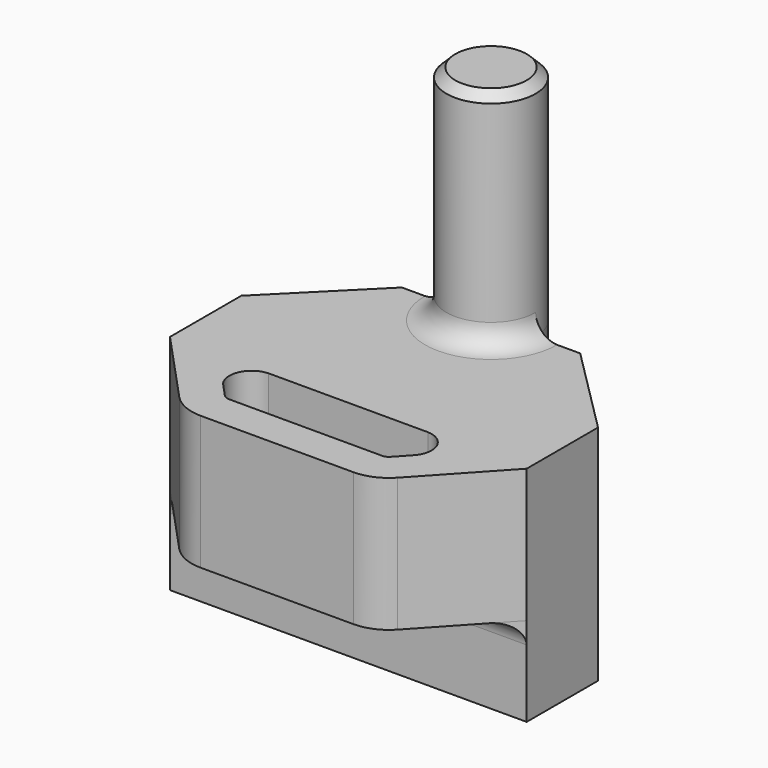
from build123d import *

# Parameters (mm, degrees)
F1_DEPTH     = 5
F2_DEPTH     = 10
F3_SIZE      = 0.2
F5_DEPTH     = 3
F6_T1_DEPTH  = 3
F6_T6_DEPTH  = 2.3418509092
F6_T12_DEPTH = 2.3418509092
F6_T16_ANGLE = 180
F6_T21_DEPTH = 2.3418509092
F6_T25_DEPTH = 5.8592538582
F6_T33_DEPTH = 5.8592538582
F6_T38_DEPTH = 2.3418509092


# Not quite as in the source:
# - a fillet or chamfer that OpenCascade refuses, or shapes differently, is made with other operations: its cross-section is extruded or revolved along the edge and cut away or added


with BuildPart() as f1:
    # F0 (on Top) → F1 (new body)
    with BuildSketch(Plane.XY):
        with BuildLine():
            Line((0, 2), (0, 0))
            Line((0, 0), (8, 0))
            Line((8, 0), (8, 2))
            Line((8, 2), (6, 4))
            Line((6, 4), (5, 4))
            ThreePointArc((5, 4), (4, 3), (3, 4))
            Line((3, 4), (2, 4))
            Line((2, 4), (0, 2))
        make_face()
        with BuildLine():
            ThreePointArc((5, 4), (4, 5), (3, 4))
            Line((3, 4), (5, 4))
        make_face()
        with BuildLine():
            Line((5, 4), (3, 4))
            ThreePointArc((3, 4), (4, 3), (5, 4))
        make_face()
    extrude(amount=F1_DEPTH)

    # F0 (on Top) → F2 (join)
    with BuildSketch(Plane.XY):
        with BuildLine():
            ThreePointArc((5, 4), (4, 5), (3, 4))
            Line((3, 4), (5, 4))
        make_face()
        with BuildLine():
            Line((5, 4), (3, 4))
            ThreePointArc((3, 4), (4, 3), (5, 4))
        make_face()
    extrude(amount=F2_DEPTH)

    # F3
    f3_edges = [f1.edges().sort_by_distance(p)[0] for p in [
        (5, 4, 10),
    ]]
    chamfer(f3_edges, length=F3_SIZE)

    # F4 (on face) → F5 (join)
    with BuildSketch(Plane.XY.offset(5)):
        with BuildLine():
            Line((1.0894362964, 0), (0, 0))
            Line((0, 0), (1.5518551177, -1.6787983581))
            ThreePointArc((1.5518551177, -1.6787983581), (1.8854295116, -1.9161873057), (2.286179834, -2))
            Line((2.286179834, -2), (5.713820166, -2))
            ThreePointArc((5.713820166, -2), (6.1145704884, -1.9161873057), (6.4481448823, -1.6787983581))
            Line((6.4481448823, -1.6787983581), (8, 0))
            Line((8, 0), (6.9105637036, 0))
            Line((6.9105637036, 0), (5.8606851097, -1.1357596721))
            ThreePointArc((5.8606851097, -1.1357596721), (5.7939702307, -1.1832374617), (5.713820166, -1.2000000007))
            Line((5.713820166, -1.2000000007), (2.286179834, -1.2000000007))
            ThreePointArc((2.286179834, -1.2000000007), (2.2060297693, -1.1832374617), (2.1393148903, -1.1357596721))
            Line((2.1393148903, -1.1357596721), (1.0894362964, 0))
        make_face()
    extrude(amount=-F5_DEPTH)

    # F6: fillet of radius 0.5 on 5 edges, made by hand

    # F6_s2 → F6_t1 (join)
    with BuildSketch(Plane.XY.offset(2)):
        with BuildLine():
            ThreePointArc((5.7668622302, 0.0004), (6.2255674394, -0.2996248388), (6.1345147512, -0.8401197793))
            Line((6.1345147512, -0.8401197793), (6.1712800033, -0.8741050071))
            ThreePointArc((6.1712800033, -0.8741050071), (6.5591576145, -0.4539093578), (6.9473289557, -0.0339852278))
            Line((6.9473289557, -0.0339852278), (6.9105637036, 0.0500667501))
            ThreePointArc((6.9105637036, 0.0500667501), (6.3387129669, 0.0500667501), (5.7668622302, 0.0504667501))
            Line((5.7668622302, 0.0504667501), (5.7668622302, 0.0004))
        make_face()
        with BuildLine():
            ThreePointArc((2.2331377698, 0.0004), (1.7744325606, -0.2996248388), (1.8654852488, -0.8401197793))
            Line((1.8654852488, -0.8401197793), (1.8287199967, -0.8741050071))
            ThreePointArc((1.8287199967, -0.8741050071), (1.4408423855, -0.4539093578), (1.0526710443, -0.0339852278))
            Line((1.0526710443, -0.0339852278), (1.0894362964, 0.0500667501))
            ThreePointArc((1.0894362964, 0.0500667501), (1.6612870331, 0.0500667501), (2.2331377698, 0.0504667501))
            Line((2.2331377698, 0.0504667501), (2.2331377698, 0.0004))
        make_face()
    extrude(amount=F6_T1_DEPTH)


with BuildPart() as f6_tool4:
    # F6_s5 → F6_t6 (new body)
    with BuildSketch(Plane.YZ.offset(8)):
        with BuildLine():
            ThreePointArc((0.0004, 1.4990343146), (-0.1464466094, 1.8535533906), (-0.5009656854, 2.0004))
            Line((-0.5009656854, 2.0004), (-0.5009656854, 2.0505365685))
            ThreePointArc((-0.5009656854, 2.0505365685), (-0.2504828427, 2.0501365685), (0, 2.0501365685))
            Line((0, 2.0501365685), (0.0501365685, 2))
            ThreePointArc((0.0501365685, 2), (0.0501365685, 1.7495171573), (0.0505365685, 1.4990343146))
            Line((0.0505365685, 1.4990343146), (0.0004, 1.4990343146))
        make_face()
    extrude(amount=-F6_T6_DEPTH)

    split(bisect_by=Plane(origin=(4.3138623121, -3.9876672942, 0), x_dir=(0, 0, 1), z_dir=(-0.7343247163, 0.6787983581, 0)), keep=Keep.TOP)

    split(bisect_by=Plane(origin=(3.7264025395, -3.4446286081, 0), x_dir=(0, 0, 1), z_dir=(0.7343247163, -0.6787983581, 0)), keep=Keep.TOP)


with BuildPart() as f1_1:
    add(f1.part)

    # F6_t3: union F6_tool4
    add(f6_tool4.part)


with BuildPart() as f6_tool10:
    # F6_s11 → F6_t12 (new body)
    with BuildSketch(Plane.YZ.offset(2.3418509092)):
        with BuildLine():
            ThreePointArc((0.0004, 1.4990343146), (-0.1464466094, 1.8535533906), (-0.5009656854, 2.0004))
            Line((-0.5009656854, 2.0004), (-0.5009656854, 2.0505365685))
            ThreePointArc((-0.5009656854, 2.0505365685), (-0.2504828427, 2.0501365685), (0, 2.0501365685))
            Line((0, 2.0501365685), (0.0501365685, 2))
            ThreePointArc((0.0501365685, 2), (0.0501365685, 1.7495171573), (0.0505365685, 1.4990343146))
            Line((0.0505365685, 1.4990343146), (0.0004, 1.4990343146))
        make_face()
    extrude(amount=-F6_T12_DEPTH)

    split(bisect_by=Plane(origin=(0, 0, 0), x_dir=(0, 0, 1), z_dir=(0.7343247163, 0.6787983581, 0)), keep=Keep.TOP)

    split(bisect_by=Plane(origin=(0.5874597726, 0.543038686, 0), x_dir=(0, 0, 1), z_dir=(-0.7343247163, -0.6787983581, 0)), keep=Keep.TOP)


with BuildPart() as f1_2:
    add(f1_1.part)

    # F6_t9: union F6_tool10
    add(f6_tool10.part)

    # F6_s15 → F6_t16 (revolve)
    with BuildSketch(Plane.XZ.offset(-4)):
        with BuildLine():
            ThreePointArc((4.9996, 5.5009656854), (5.1464466094, 5.1464466094), (5.5009656854, 4.9996))
            Line((5.5009656854, 4.9996), (5.5009656854, 4.9494634315))
            ThreePointArc((5.5009656854, 4.9494634315), (5.2504828427, 4.9498634315), (5, 4.9498634315))
            Line((5, 4.9498634315), (4.9498634315, 5))
            ThreePointArc((4.9498634315, 5), (4.9498634315, 5.2504828427), (4.9494634315, 5.5009656854))
            Line((4.9494634315, 5.5009656854), (4.9996, 5.5009656854))
        make_face()
    revolve(axis=Axis((4, 4, 5), (0, 0, -1)), revolution_arc=F6_T16_ANGLE)


with BuildPart() as f6_tool19:
    # F6_s20 → F6_t21 (new body)
    with BuildSketch(Plane.YZ.offset(8)):
        with BuildLine():
            ThreePointArc((0.0004, 1.4990343146), (-0.1464466094, 1.8535533906), (-0.5009656854, 2.0004))
            Line((-0.5009656854, 2.0004), (-0.5009656854, 2.0505365685))
            ThreePointArc((-0.5009656854, 2.0505365685), (-0.2504828427, 2.0501365685), (0, 2.0501365685))
            Line((0, 2.0501365685), (0.0501365685, 2))
            ThreePointArc((0.0501365685, 2), (0.0501365685, 1.7495171573), (0.0505365685, 1.4990343146))
            Line((0.0505365685, 1.4990343146), (0.0004, 1.4990343146))
        make_face()
    extrude(amount=-F6_T21_DEPTH)

    split(bisect_by=Plane(origin=(3.7264025395, -3.4446286081, 0), x_dir=(0, 0, 1), z_dir=(-0.7343247163, 0.6787983581, 0)), keep=Keep.TOP)


with BuildPart() as f6_tool23:
    # F6_s24 → F6_t25 (new body)
    with BuildSketch(Plane.XY.offset(5)):
        with BuildLine():
            ThreePointArc((5.7668622302, 0.0004), (6.2255674394, -0.2996248388), (6.1345147512, -0.8401197793))
            Line((6.1345147512, -0.8401197793), (6.1712800033, -0.8741050071))
            ThreePointArc((6.1712800033, -0.8741050071), (6.5591576145, -0.4539093578), (6.9473289557, -0.0339852278))
            Line((6.9473289557, -0.0339852278), (6.9105637036, 0.0500667501))
            ThreePointArc((6.9105637036, 0.0500667501), (6.3387129669, 0.0500667501), (5.7668622302, 0.0504667501))
            Line((5.7668622302, 0.0504667501), (5.7668622302, 0.0004))
        make_face()
    extrude(amount=-F6_T25_DEPTH)

    split(bisect_by=Plane.XY, keep=Keep.TOP)

    split(bisect_by=Plane.XY.offset(2), keep=Keep.BOTTOM)


with BuildPart() as f6_tool19_1:
    add(f6_tool19.part)

    # F6_t28: intersect F6_tool23
    add(f6_tool23.part, mode=Mode.INTERSECT)


with BuildPart() as f1_3:
    add(f1_2.part)

    # F6_t17: union F6_tool19
    add(f6_tool19_1.part)


with BuildPart() as f6_tool31:
    # F6_s32 → F6_t33 (new body)
    with BuildSketch(Plane.XY.offset(5)):
        with BuildLine():
            ThreePointArc((2.2331377698, 0.0004), (1.7744325606, -0.2996248388), (1.8654852488, -0.8401197793))
            Line((1.8654852488, -0.8401197793), (1.8287199967, -0.8741050071))
            ThreePointArc((1.8287199967, -0.8741050071), (1.4408423855, -0.4539093578), (1.0526710443, -0.0339852278))
            Line((1.0526710443, -0.0339852278), (1.0894362964, 0.0500667501))
            ThreePointArc((1.0894362964, 0.0500667501), (1.6612870331, 0.0500667501), (2.2331377698, 0.0504667501))
            Line((2.2331377698, 0.0504667501), (2.2331377698, 0.0004))
        make_face()
    extrude(amount=-F6_T33_DEPTH)

    split(bisect_by=Plane.XY, keep=Keep.TOP)

    split(bisect_by=Plane.XY.offset(2), keep=Keep.BOTTOM)


with BuildPart() as f6_tool36:
    # F6_s37 → F6_t38 (new body)
    with BuildSketch(Plane.YZ.offset(2.3418509092)):
        with BuildLine():
            ThreePointArc((0.0004, 1.4990343146), (-0.1464466094, 1.8535533906), (-0.5009656854, 2.0004))
            Line((-0.5009656854, 2.0004), (-0.5009656854, 2.0505365685))
            ThreePointArc((-0.5009656854, 2.0505365685), (-0.2504828427, 2.0501365685), (0, 2.0501365685))
            Line((0, 2.0501365685), (0.0501365685, 2))
            ThreePointArc((0.0501365685, 2), (0.0501365685, 1.7495171573), (0.0505365685, 1.4990343146))
            Line((0.0505365685, 1.4990343146), (0.0004, 1.4990343146))
        make_face()
    extrude(amount=-F6_T38_DEPTH)

    split(bisect_by=Plane(origin=(0.5874597726, 0.543038686, 0), x_dir=(0, 0, 1), z_dir=(0.7343247163, 0.6787983581, 0)), keep=Keep.TOP)


with BuildPart() as f6_tool31_1:
    add(f6_tool31.part)

    # F6_t40: intersect F6_tool36
    add(f6_tool36.part, mode=Mode.INTERSECT)


with BuildPart() as f1_4:
    add(f1_3.part)

    # F6_t29: union F6_tool31
    add(f6_tool31_1.part)


solid = f1_4.part
